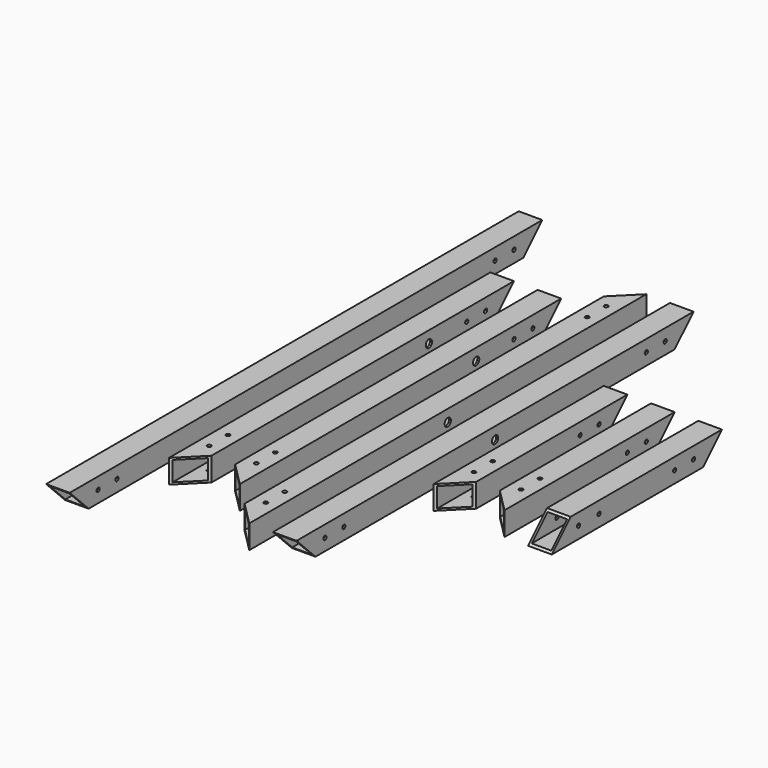
from build123d import *

# Parameters (mm, degrees)
F0_W      = 38.1
F0_H      = 38.1
F0_W_2    = 31.75
F0_H_2    = 31.75
F1_DEPTH  = 457.2
F2_R      = 6.35
F2_R_2    = 3.175
F3_DEPTH  = 76.2
F4_W      = 38.1
F4_H      = 38.1
F4_W_2    = 31.75
F4_H_2    = 31.75
F5_DEPTH  = 457.2
F6_R      = 6.35
F7_DEPTH  = 38.101
F8_R      = 3.175
F9_DEPTH  = 38.101
F10_W     = 38.1
F10_H     = 38.1
F10_W_2   = 31.75
F10_H_2   = 31.75
F11_DEPTH = 228.6
F12_W     = 38.1
F12_H     = 38.1
F12_W_2   = 31.75
F12_H_2   = 31.75
F13_DEPTH = 228.6
F14_R     = 3.175
F15_DEPTH = 247.651
F16_R     = 3.175
F17_DEPTH = 38.101
F18_R     = 3.175
F19_DEPTH = 38.101
F20_R     = 3.175
F21_DEPTH = 342.901
F22_W     = 38.1
F22_H     = 38.1
F22_W_2   = 31.75
F22_H_2   = 31.75
F23_DEPTH = 355.6
F24_DEPTH = 508
F25_R     = 3.175
F25_R_2   = 6.35
F26_DEPTH = 190.501
F27_R     = 3.175
F28_DEPTH = 38.101
F29_R     = 3.175
F30_DEPTH = 38.101
F31_R     = 3.175
F32_DEPTH = 38.101
F33_R     = 3.175
F34_DEPTH = 571.501


with BuildPart() as f1:
    # F0 (on Front) → F1 (new body, symmetric)
    with BuildSketch(Plane.XZ):
        Rectangle(F0_W, F0_H)
        Rectangle(F0_W_2, F0_H_2, mode=Mode.SUBTRACT)
    extrude(amount=F1_DEPTH, both=True)

    # F2 (on Right) → F3 (cut, symmetric)
    with BuildSketch(Plane.YZ):
        Circle(F2_R)
        Polygon((-304.8, -76.2), (-381, 0), (-457.2, 76.2), (-558.8, 76.2), (-558.8, -76.2), align=None)
        with Locations((-304.8, 0)):
            Circle(F2_R_2)
        with Locations((-342.9, 0)):
            Circle(F2_R_2)
        with Locations((342.9, 0)):
            Circle(F2_R_2)
        with Locations((304.8, 0)):
            Circle(F2_R_2)
        Polygon((304.8, -76.2), (558.8, -76.2), (558.8, 76.2), (457.2, 76.2), (381, 0), align=None)
    extrude(amount=F3_DEPTH, both=True, mode=Mode.SUBTRACT)


with BuildPart() as f5:
    # F4 (on Front) → F5 (new body, symmetric)
    with BuildSketch(Plane.XZ):
        with Locations((-76.2, 0)):
            Rectangle(F4_W, F4_H)
        with Locations((-76.2, 0)):
            Rectangle(F4_W_2, F4_H_2, mode=Mode.SUBTRACT)
    extrude(amount=F5_DEPTH, both=True)

    # F6 (on face) → F7 (cut, through all)
    with BuildSketch(Plane.YZ.offset(-57.15)):
        Circle(F6_R)
    extrude(amount=-F7_DEPTH, mode=Mode.SUBTRACT)

    # F8 (on face) → F9 (cut, through all)
    with BuildSketch(Plane.XY.offset(19.05)):
        Polygon((-127, 330.2), (-76.2, 381), (-25.4, 431.8), (-25.4, 533.4), (-127, 533.4), align=None)
        with Locations((-76.2, 342.9)):
            Circle(F8_R)
        with Locations((-76.2, 304.8)):
            Circle(F8_R)
        with Locations((-76.2, -304.8)):
            Circle(F8_R)
        with Locations((-76.2, -342.9)):
            Circle(F8_R)
        Polygon((-25.4, -431.8), (-76.2, -381), (-127, -330.2), (-127, -533.4), (-25.4, -533.4), align=None)
    extrude(amount=-F9_DEPTH, mode=Mode.SUBTRACT)


with BuildPart() as f11:
    # F10 (on Front) → F11 (new body, symmetric)
    with BuildSketch(Plane.XZ):
        with Locations((76.2, 0)):
            Rectangle(F10_W, F10_H)
        with Locations((76.2, 0)):
            Rectangle(F10_W_2, F10_H_2, mode=Mode.SUBTRACT)
    extrude(amount=F11_DEPTH, both=True)


with BuildPart() as f13:
    # F12 (on Front) → F13 (new body, symmetric)
    with BuildSketch(Plane.XZ):
        with Locations((152.4, 0)):
            Rectangle(F12_W, F12_H)
        with Locations((152.4, 0)):
            Rectangle(F12_W_2, F12_H_2, mode=Mode.SUBTRACT)
    extrude(amount=F13_DEPTH, both=True)


with BuildPart() as f13b:
    # F12 (on Front) → F13, piece 2 (new body, symmetric)
    with BuildSketch(Plane.XZ):
        with Locations((228.6, 0)):
            Rectangle(F12_W, F12_H)
        with Locations((228.6, 0)):
            Rectangle(F12_W_2, F12_H_2, mode=Mode.SUBTRACT)
    extrude(amount=F13_DEPTH, both=True)


with BuildPart() as f15_tool:
    # F14 (on Right) → F15 (new body, through all)
    with BuildSketch(Plane.YZ):
        Polygon((203.2, 50.8), (152.4, 0), (101.6, -50.8), (304.8, -50.8), (304.8, 50.8), align=None)
        with Locations((76.2, 0)):
            Circle(F14_R)
        with Locations((114.3, 0)):
            Circle(F14_R)
    extrude(amount=F15_DEPTH)


with BuildPart() as f11_1:
    add(f11.part)

    # F15: cut by f15_tool
    add(f15_tool.part, mode=Mode.SUBTRACT)

    # F16 (on face) → F17 (cut, through all)
    with BuildSketch(Plane.XY.offset(19.05)):
        Polygon((127, -101.6), (76.2, -152.4), (25.4, -203.2), (25.4, -304.8), (127, -304.8), align=None)
        with Locations((76.2, -76.2)):
            Circle(F16_R)
        with Locations((76.2, -114.3)):
            Circle(F16_R)
    extrude(amount=-F17_DEPTH, mode=Mode.SUBTRACT)


with BuildPart() as f13_1:
    add(f13.part)

    # F15: cut by f15_tool
    add(f15_tool.part, mode=Mode.SUBTRACT)

    # F18 (on face) → F19 (cut, through all)
    with BuildSketch(Plane.XY.offset(19.05)):
        Polygon((203.2, -203.2), (152.4, -152.4), (101.6, -101.6), (101.6, -304.8), (203.2, -304.8), align=None)
        with Locations((152.4, -76.2)):
            Circle(F18_R)
        with Locations((152.4, -114.3)):
            Circle(F18_R)
    extrude(amount=-F19_DEPTH, mode=Mode.SUBTRACT)


with BuildPart() as f13b_1:
    add(f13b.part)

    # F15: cut by f15_tool
    add(f15_tool.part, mode=Mode.SUBTRACT)

    # F20 (on face) → F21 (cut, through all)
    with BuildSketch(Plane.YZ.offset(247.65)):
        Polygon((-152.4, 0), (-101.6, 50.8), (-304.8, 50.8), (-304.8, -50.8), (-203.2, -50.8), align=None)
        with Locations((-117.475, 0)):
            Circle(F20_R)
        with Locations((-76.2, 0)):
            Circle(F20_R)
    extrude(amount=-F21_DEPTH, mode=Mode.SUBTRACT)


with BuildPart() as f23:
    # F22 (on Front) → F23 (new body, symmetric)
    with BuildSketch(Plane.XZ):
        with Locations((-152.4, 0)):
            Rectangle(F22_W, F22_H)
        with Locations((-152.4, 0)):
            Rectangle(F22_W_2, F22_H_2, mode=Mode.SUBTRACT)
    extrude(amount=F23_DEPTH, both=True)


with BuildPart() as f23b:
    # F22 (on Front) → F23, piece 2 (new body, symmetric)
    with BuildSketch(Plane.XZ):
        with Locations((-228.6, 0)):
            Rectangle(F22_W, F22_H)
        with Locations((-228.6, 0)):
            Rectangle(F22_W_2, F22_H_2, mode=Mode.SUBTRACT)
    extrude(amount=F23_DEPTH, both=True)


with BuildPart() as f24:
    # F22 (on Front) → F24 (new body, symmetric)
    with BuildSketch(Plane.XZ):
        with Locations((-304.8, 0)):
            Rectangle(F22_W, F22_H)
        with Locations((-304.8, 0)):
            Rectangle(F22_W_2, F22_H_2, mode=Mode.SUBTRACT)
    extrude(amount=F24_DEPTH, both=True)

    # F27 (on face) → F28 (cut, through all)
    with BuildSketch(Plane.YZ.offset(-285.75)):
        Polygon((508, 50.8), (457.2, 0), (406.4, -50.8), (609.6, -50.8), (609.6, 50.8), align=None)
        with Locations((381, 0)):
            Circle(F27_R)
        with Locations((419.1, 0)):
            Circle(F27_R)
    extrude(amount=-F28_DEPTH, mode=Mode.SUBTRACT)

    # F33 (on face) → F34 (cut, through all)
    with BuildSketch(Plane(origin=(-323.85, 0, 0), x_dir=(0, -1, 0), z_dir=(-1, 0, 0))):
        Polygon((508, 50.7999994945), (457.2, -5.055e-07), (406.4, -50.8000005055), (609.6, -50.8000005055), (609.6, 50.7999994945), align=None)
        with Locations((381, -5.055e-07)):
            Circle(F33_R)
        with Locations((419.1, -5.055e-07)):
            Circle(F33_R)
    extrude(amount=-F34_DEPTH, mode=Mode.SUBTRACT)


with BuildPart() as f26_tool:
    # F25 (on face) → F26 (new body, through all)
    with BuildSketch(Plane.YZ.offset(-133.35)):
        Polygon((355.6, 50.8), (304.8, 0), (254, -50.8), (457.2, -50.8), (457.2, 50.8), align=None)
        with Locations((228.6, 0)):
            Circle(F25_R)
        with Locations((266.7, 0)):
            Circle(F25_R)
        with Locations((152.4, 0)):
            Circle(F25_R_2)
    extrude(amount=-F26_DEPTH)


with BuildPart() as f23_1:
    add(f23.part)

    # F26: cut by f26_tool
    add(f26_tool.part, mode=Mode.SUBTRACT)

    # F29 (on face) → F30 (cut, through all)
    with BuildSketch(Plane.XY.offset(19.05)):
        Polygon((-101.6, -355.6), (-152.4, -304.8), (-203.2, -254), (-203.2, -457.2), (-101.6, -457.2), align=None)
        with Locations((-152.4, -228.6)):
            Circle(F29_R)
        with Locations((-152.4, -266.7)):
            Circle(F29_R)
    extrude(amount=-F30_DEPTH, mode=Mode.SUBTRACT)


with BuildPart() as f23b_1:
    add(f23b.part)

    # F26: cut by f26_tool
    add(f26_tool.part, mode=Mode.SUBTRACT)

    # F31 (on face) → F32 (cut, through all)
    with BuildSketch(Plane.XY.offset(19.05)):
        Polygon((-177.8, -254), (-228.6, -304.8), (-279.4, -355.6), (-279.4, -457.2), (-177.8, -457.2), align=None)
        with Locations((-228.6, -228.6)):
            Circle(F31_R)
        with Locations((-228.6, -266.7)):
            Circle(F31_R)
    extrude(amount=-F32_DEPTH, mode=Mode.SUBTRACT)


solid = Compound([f1.part, f5.part, f11_1.part, f13_1.part, f13b_1.part, f24.part, f23_1.part, f23b_1.part])
